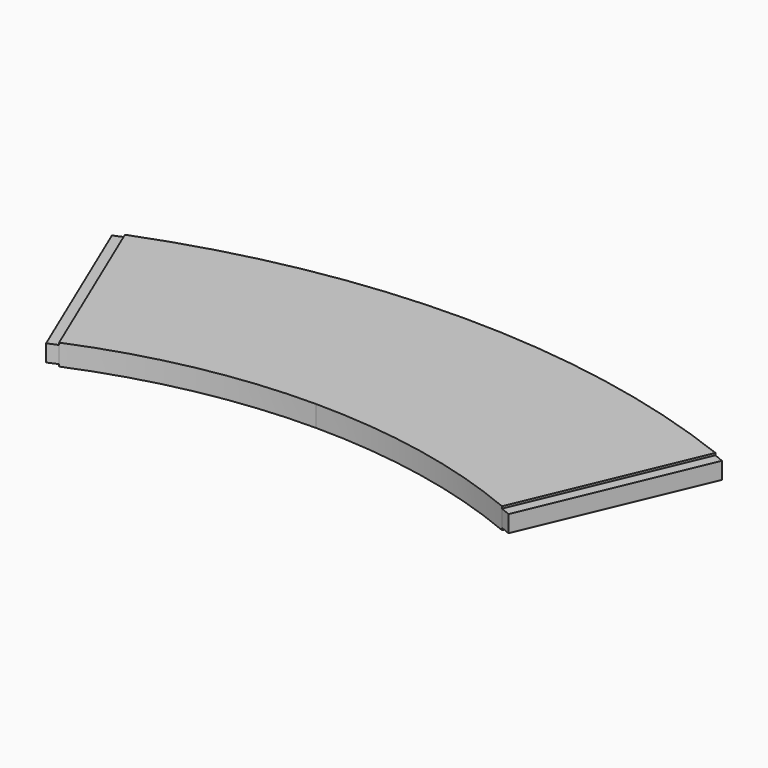
from build123d import *

# Parameters (mm, degrees)
F1_DEPTH = 10
F2_W     = 89.8676701995
F2_H     = 8
F3_DEPTH = 5
F4_W     = 89.8676701995
F4_H     = 8
F5_DEPTH = 5


# Not quite as in the source:
# - a feature names something its author has since deleted; it is built from what else it names


with BuildPart() as f1:
    # F0 (on Top) → F1 (new body)
    with BuildSketch(Plane.XY):
        with BuildLine():
            Line((0, 0), (-140, 0))
            Line((-140, 0), (-105, -82.771964741))
            ThreePointArc((-105, -82.771964741), (-53.5397048927, -67.0734402774), (0, -61.771964741))
            Line((0, -61.771964741), (0, 0))
        make_face()
        with BuildLine():
            Line((140, 0), (0, 0))
            Line((0, 0), (0, -61.771964741))
            ThreePointArc((0, -61.771964741), (53.5397048927, -67.0734402774), (105, -82.771964741))
            Line((105, -82.771964741), (140, 0))
        make_face()
        with BuildLine():
            ThreePointArc((0, 26.228035259), (-71.217817001, 19.6144809107), (-140, 0))
            Line((-140, 0), (0, 0))
            Line((0, 0), (0, 26.228035259))
        make_face()
        with BuildLine():
            Line((0, 26.228035259), (0, 0))
            Line((0, 0), (140, 0))
            ThreePointArc((140, 0), (71.217817001, 19.6144809107), (0, 26.228035259))
        make_face()
    extrude(amount=F1_DEPTH)

    # F2 (on face) → F3 (join)
    with BuildSketch(Plane(origin=(118.7647607356, -50.2194993045, 0), x_dir=(0.3894615263, 0.9210427349, 0), z_dir=(0.9210427349, -0.3894615263, 0))):
        with Locations((9.5907785808, 5)):
            Rectangle(F2_W, F2_H)
    extrude(amount=F3_DEPTH)

    # F4 (on face) → F5 (join)
    with BuildSketch(Plane(origin=(-118.7647607356, -50.2194993045, 0), x_dir=(0.3894615263, -0.9210427349, 0), z_dir=(-0.9210427349, -0.3894615263, 0))):
        with Locations((-9.5907785808, 5)):
            Rectangle(F4_W, F4_H)
    extrude(amount=F5_DEPTH)


solid = f1.part
